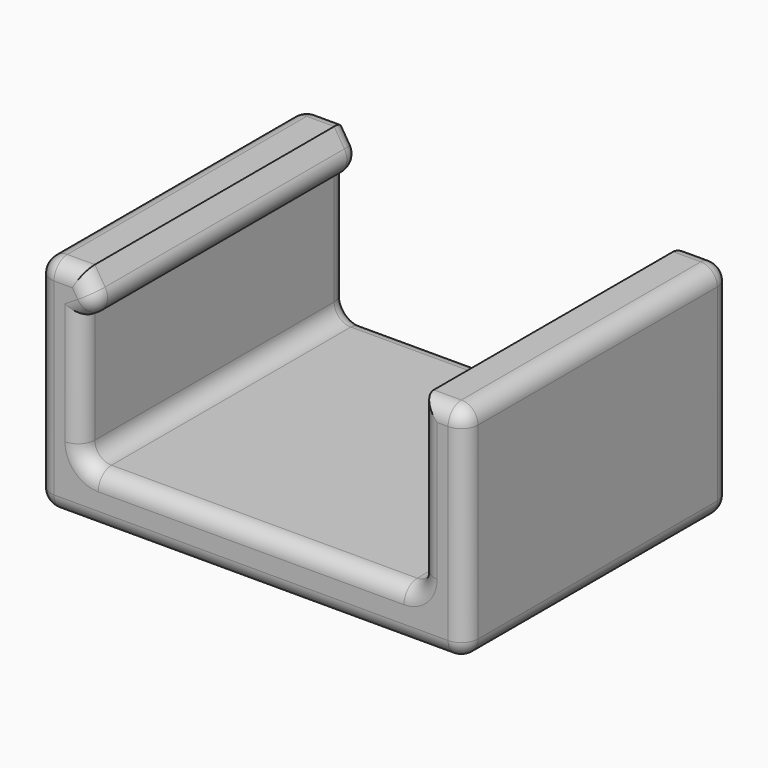
from build123d import *

# Parameters (mm, degrees)
F1_DEPTH = 30
F2_R     = 1.5


# Not quite as in the source:
# - a feature names something its author has since deleted; it is built from what else it names


with BuildPart() as f1:
    # F0 (on Front) → F1 (new body)
    with BuildSketch(Plane.XZ):
        with BuildLine():
            ThreePointArc((-50.6280393004, 55.2302640676), (-51.6886994722, 54.7909242394), (-52.1280393004, 53.7302640676))
            Line((-52.1280393004, 53.7302640676), (-52.1280393004, 36.7302640676))
            ThreePointArc((-52.1280393004, 36.7302640676), (-51.6886994722, 35.6696038959), (-50.6280393004, 35.2302640676))
            Line((-50.6280393004, 35.2302640676), (-15.0573858261, 35.2302640676))
            ThreePointArc((-15.0573858261, 35.2302640676), (-13.9967256543, 35.6696038959), (-13.5573858261, 36.7302640676))
            Line((-13.5573858261, 36.7302640676), (-13.5573858261, 53.7302640676))
            ThreePointArc((-13.5573858261, 53.7302640676), (-13.9967256543, 54.7909242394), (-15.0573858261, 55.2302640676))
            Line((-15.0573858261, 55.2302640676), (-17.5427125633, 55.2302640676))
            Line((-17.5427125633, 55.2302640676), (-17.5427125633, 41.2777487338))
            ThreePointArc((-17.5427125633, 41.2777487338), (-17.9820523915, 40.217088562), (-19.0427125633, 39.7777487338))
            Line((-19.0427125633, 39.7777487338), (-46.6427125633, 39.7777487338))
            ThreePointArc((-46.6427125633, 39.7777487338), (-47.7033727351, 40.217088562), (-48.1427125633, 41.2777487338))
            Line((-48.1427125633, 41.2777487338), (-48.1427125633, 51.408215398))
            Line((-48.1427125633, 51.408215398), (-47.7003021707, 51.6838852273))
            ThreePointArc((-47.7003021707, 51.6838852273), (-47.032442186, 52.6176852731), (-47.2204902066, 53.7502299418))
            Line((-47.2204902066, 53.7502299418), (-48.1427125633, 55.2302640676))
            Line((-48.1427125633, 55.2302640676), (-50.6280393004, 55.2302640676))
        make_face()
    extrude(amount=F1_DEPTH)

    # F2
    f2_edges = [f1.edges().sort_by_distance(p)[0] for p in [
        (-49.385376, -30, 55.230264),
        (-51.688699, -30, 54.790924),
        (-52.128039, -30, 45.230264),
        (-51.688699, -30, 35.669604),
        (-32.842713, -30, 35.230264),
        (-13.996726, -30, 35.669604),
        (-13.557386, -30, 45.230264),
        (-13.996726, -30, 54.790924),
        (-16.300049, -30, 55.230264),
        (-17.542713, -30, 48.254006),
        (-17.982052, -30, 40.217089),
        (-32.842713, -30, 39.777749),
        (-47.703373, -30, 40.217089),
        (-48.142713, -30, 46.342982),
        (-47.921507, -30, 51.54605),
        (-47.032442, -30, 52.617685),
        (-47.681601, -30, 54.490247),
        (-49.385376, 0, 55.230264),
        (-51.688699, 0, 54.790924),
        (-52.128039, 0, 45.230264),
        (-51.688699, 0, 35.669604),
        (-32.842713, 0, 35.230264),
        (-13.996726, 0, 35.669604),
        (-13.557386, 0, 45.230264),
        (-13.996726, 0, 54.790924),
        (-16.300049, 0, 55.230264),
        (-17.542713, 0, 48.254006),
        (-17.982052, 0, 40.217089),
        (-32.842713, 0, 39.777749),
        (-47.703373, 0, 40.217089),
        (-48.142713, 0, 46.342982),
        (-47.921507, 0, 51.54605),
        (-47.032442, 0, 52.617685),
        (-47.681601, 0, 54.490247),
    ]]
    fillet(f2_edges, radius=F2_R)


solid = f1.part
